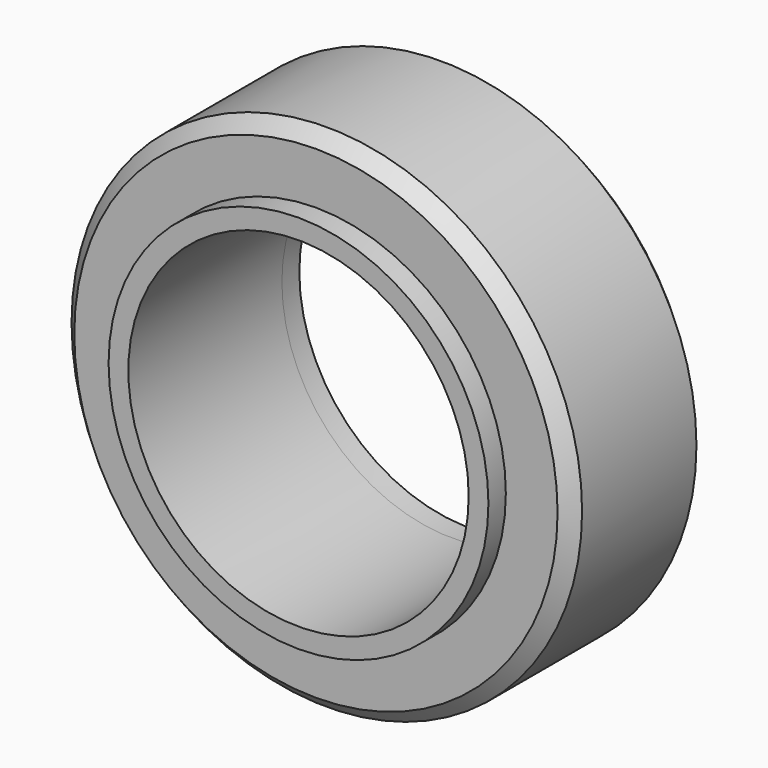
from build123d import *

# Parameters (mm, degrees)
F0_R     = 4.7625
F0_R_2   = 3.175
F1_DEPTH = 3.175
F2_R     = 3.5433
F2_R_2   = 3.175
F3_DEPTH = 0.4064
F4_R     = 3.5433
F4_R_2   = 3.175
F5_DEPTH = 0.4064
F6_SIZE  = 0.254


with BuildPart() as f1:
    # F0 (on Front) → F1 (new body)
    with BuildSketch(Plane.XZ):
        Circle(F0_R)
        Circle(F0_R_2, mode=Mode.SUBTRACT)
    extrude(amount=F1_DEPTH)

    # F2 (on face) → F3 (join)
    with BuildSketch(Plane.XZ.offset(3.175)):
        Circle(F2_R)
        Circle(F2_R_2, mode=Mode.SUBTRACT)
    extrude(amount=F3_DEPTH)

    # F4 (on face) → F5 (join)
    with BuildSketch(Plane(origin=(0, 0, 0), x_dir=(-1, 0, 0), z_dir=(0, 1, 0))):
        Circle(F4_R)
        Circle(F4_R_2, mode=Mode.SUBTRACT)
    extrude(amount=F5_DEPTH)

    # F6
    f6_edges = [f1.edges().sort_by_distance(p)[0] for p in [
        (-4.7625, -3.175, 0),
        (-4.7625, 0, 0),
    ]]
    chamfer(f6_edges, length=F6_SIZE)


solid = f1.part
